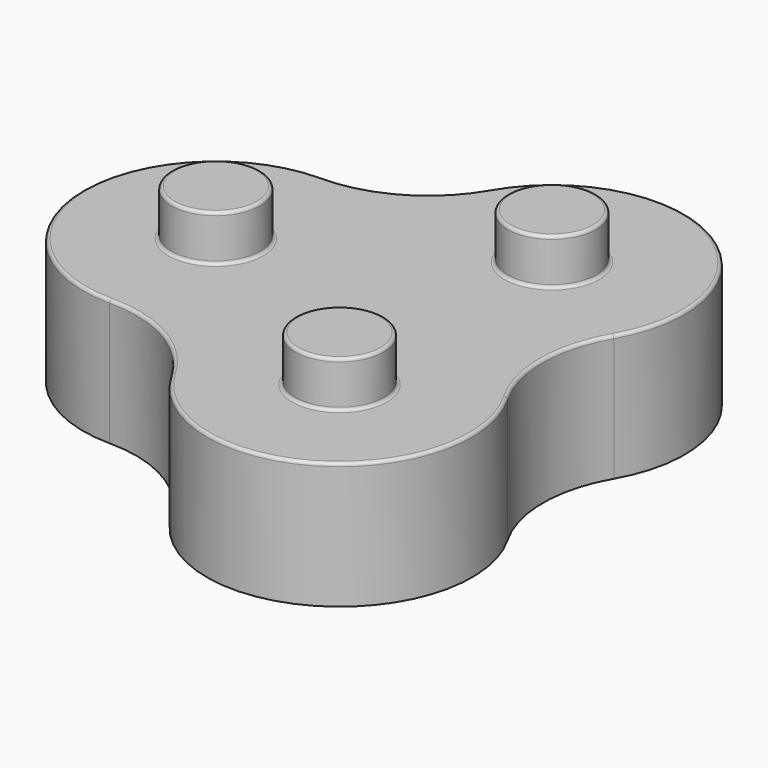
from build123d import *

# Parameters (mm, degrees)
F4_R     = 7.9
F5_DEPTH = 20
F6_DEPTH = 10
F7_R     = 7
F8_DEPTH = 7.3
F9_R     = 0.5


# Not quite as in the source:
# - a feature names something its author has since deleted; it is built from what else it names


with BuildPart() as f5:
    # F4 (on Top) → F5 (new body)
    with BuildSketch(Plane.XY):
        with BuildLine():
            ThreePointArc((18.1865334795, 10.5), (15.3730669589, 21), (18.1865334795, 31.5))
            ThreePointArc((18.1865334795, 31.5), (10.5, 60.1865334795), (-18.1865334795, 52.5))
            ThreePointArc((-18.1865334795, 52.5), (-25.8730669589, 44.8134665205), (-36.3730669589, 42))
            ThreePointArc((-36.3730669589, 42), (-57.3730669589, 21), (-36.3730669589, 0))
            ThreePointArc((-36.3730669589, 0), (-25.8730669589, -2.8134665205), (-18.1865334795, -10.5))
            ThreePointArc((-18.1865334795, -10.5), (10.5, -18.1865334795), (18.1865334795, 10.5))
        make_face()
        Circle(F4_R, mode=Mode.SUBTRACT)
        with Locations((-36.3730669589, 21)):
            Circle(F4_R, mode=Mode.SUBTRACT)
        with Locations((0, 42)):
            Circle(F4_R, mode=Mode.SUBTRACT)
        with Locations((0, 42)):
            Circle(F4_R)
        Circle(F4_R)
        with Locations((-36.3730669589, 21)):
            Circle(F4_R)
    extrude(amount=F5_DEPTH)

    # F4 (on Top) → F6 (cut)
    with BuildSketch(Plane.XY):
        with Locations((0, 42)):
            Circle(F4_R)
        Circle(F4_R)
        with Locations((-36.3730669589, 21)):
            Circle(F4_R)
    extrude(amount=F6_DEPTH, mode=Mode.SUBTRACT)

    # F7 (on face) → F8 (join)
    with BuildSketch(Plane.XY.offset(20)):
        Circle(F7_R)
        with Locations((0, 42)):
            Circle(F7_R)
        with Locations((-36.3730669589, 21)):
            Circle(F7_R)
    extrude(amount=F8_DEPTH)

    # F9
    f9_edges = [f5.edges().sort_by_distance(p)[0] for p in [
        (-7, 0, 27.3),
        (-7.9, 42, 0),
        (-7.9, 42, 10),
        (-7.9, 0, 0),
        (-7.9, 0, 10),
        (-7, 42, 27.3),
        (-7, 42, 20),
        (10.5, 60.186533, 20),
        (-43.373067, 21, 20),
        (-43.373067, 21, 27.3),
        (-28.473067, 21, 5),
        (-44.273067, 21, 0),
        (-44.273067, 21, 10),
        (-7, 0, 20),
    ]]
    fillet(f9_edges, radius=F9_R)


solid = f5.part
